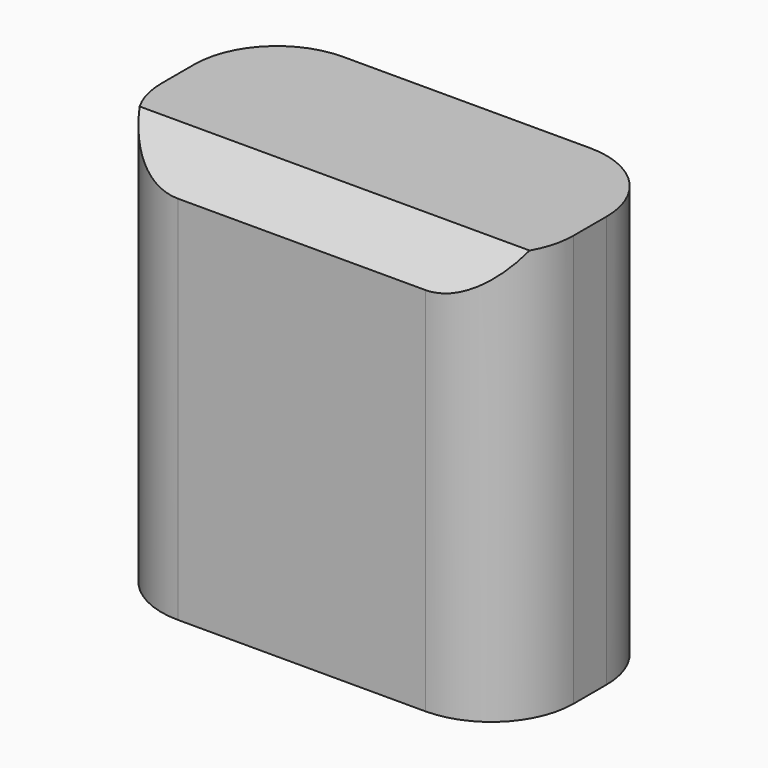
from build123d import *

# Parameters (mm, degrees)
F0_W        = 25.4
F0_H        = 12.7
F1_DEPTH    = 25.4
F2_R        = 5.08
F3_T1_DEPTH = 28.3041495789


# Not quite as in the source:
# - a fillet or chamfer that OpenCascade refuses, or shapes differently, is made with other operations: its cross-section is extruded or revolved along the edge and cut away or added


with BuildPart() as f1:
    # F0 (on Top) → F1 (new body)
    with BuildSketch(Plane.XY):
        with Locations((-7.3743816465, 11.2398102205)):
            Rectangle(F0_W, F0_H)
    extrude(amount=F1_DEPTH)

    # F2
    f2_edges = [f1.edges().sort_by_distance(p)[0] for p in [
        (5.325618, 4.88981, 12.7),
        (5.325618, 17.58981, 12.7),
        (-20.074382, 17.58981, 12.7),
        (-20.074382, 4.88981, 12.7),
    ]]
    fillet(f2_edges, radius=F2_R)

    # F3: chamfer of 2.54 on 1 edges, made by hand

    # F3_s2 → F3_t1 (cut)
    with BuildSketch(Plane.YZ.offset(-21.5264564359)):
        Polygon((7.4298102205, 25.4), (4.8898102205, 22.86), (4.8898102205, 25.4), align=None)
    extrude(amount=F3_T1_DEPTH, mode=Mode.SUBTRACT)


solid = f1.part
